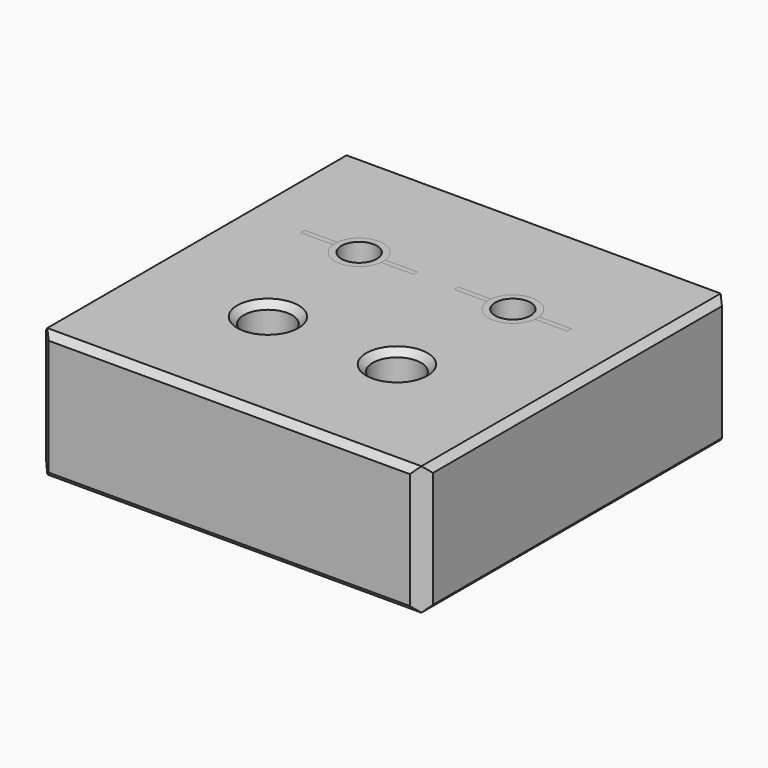
from build123d import *

# Parameters (mm, degrees)
F0_W        = 38.1
F0_H        = 76.2
F0_R        = 4.7625
F1_DEPTH    = 25.4
F2_SIZE     = 2.54
F3_SIZE     = 1.26999
F4_T1_DEPTH = 78.9220847894
F4_T3_DEPTH = 76.5265699849
F0_R_2      = 3.4925
F5_DEPTH    = 22.225
F6_DEPTH    = 22.225
F7_DEPTH    = 22.225
F8_SIZE     = 0.762
F8_2_SIZE   = 0.762
F9_SIZE2    = 1.6497783942
F9_SIZE     = 0.9525


# Not quite as in the source:
# - a fillet or chamfer that OpenCascade refuses, or shapes differently, is made with other operations: its cross-section is extruded or revolved along the edge and cut away or added
# - a fillet or chamfer is up to 0.001 mm smaller than in the source, because OpenCascade refuses the exact size


with BuildPart() as f1:
    # F0 (on Top) → F1 (new body)
    with BuildSketch(Plane.XY):
        with Locations((-19.05, 0)):
            Rectangle(F0_W, F0_H)
        with Locations((-12.7, -12.7)):
            Circle(F0_R, mode=Mode.SUBTRACT)
        with BuildLine():
            ThreePointArc((-19.8702153916, 13.3115481797), (-15.134886232, 17.5660481797), (-10.3995570724, 13.3115481797))
            Line((-10.3995570724, 13.3115481797), (-4.022386232, 13.3115481797))
            Line((-4.022386232, 13.3115481797), (-4.022386232, 12.2955481797))
            Line((-4.022386232, 12.2955481797), (-10.3995570724, 12.2955481797))
            ThreePointArc((-10.3995570724, 12.2955481797), (-15.134886232, 8.0410481797), (-19.8702153916, 12.2955481797))
            Line((-19.8702153916, 12.2955481797), (-26.247386232, 12.2955481797))
            Line((-26.247386232, 12.2955481797), (-26.247386232, 13.3115481797))
            Line((-26.247386232, 13.3115481797), (-19.8702153916, 13.3115481797))
        make_face(mode=Mode.SUBTRACT)
        with Locations((19.05, 0)):
            Rectangle(F0_W, F0_H)
        with Locations((12.7, -12.7)):
            Circle(F0_R, mode=Mode.SUBTRACT)
        with BuildLine():
            ThreePointArc((10.3995570724, 13.3115481797), (15.134886232, 17.5660481797), (19.8702153916, 13.3115481797))
            Line((19.8702153916, 13.3115481797), (26.247386232, 13.3115481797))
            Line((26.247386232, 13.3115481797), (26.247386232, 12.2955481797))
            Line((26.247386232, 12.2955481797), (19.8702153916, 12.2955481797))
            ThreePointArc((19.8702153916, 12.2955481797), (15.134886232, 8.0410481797), (10.3995570724, 12.2955481797))
            Line((10.3995570724, 12.2955481797), (4.022386232, 12.2955481797))
            Line((4.022386232, 12.2955481797), (4.022386232, 13.3115481797))
            Line((4.022386232, 13.3115481797), (10.3995570724, 13.3115481797))
        make_face(mode=Mode.SUBTRACT)
    extrude(amount=-F1_DEPTH)

    # F2
    f2_edges = [f1.edges().sort_by_distance(p)[0] for p in [
        (38.1, -38.1, -12.7),
        (38.1, 38.1, -12.7),
        (-38.1, -38.1, -12.7),
    ]]
    chamfer(f2_edges, length=F2_SIZE)

    # F3 (size 1.27 in the source; OpenCascade refuses exactly that, so slightly less here)
    f3_edges = [f1.edges().sort_by_distance(p)[0] for p in [
        (0, -38.1, 0),
        (-1.27, 38.1, 0),
        (38.1, 0, 0),
        (38.1, 0, -25.4),
        (0, -38.1, -25.4),
        (-1.27, 38.1, -25.4),
        (-38.1, 1.27, -25.4),
    ]]
    chamfer(f3_edges, length=F3_SIZE)

    # F4: chamfer of 1.27 on 4 edges, made by hand

    # F4_s2 → F4_t1 (cut)
    with BuildSketch(Plane.XZ.offset(-40.0960473947)):
        Polygon((-38.1, -1.27), (-36.83, 0), (-38.1, 0), align=None)
    extrude(amount=F4_T1_DEPTH, mode=Mode.SUBTRACT)

    # F4_s4 → F4_t3 (cut)
    with BuildSketch(Plane.XZ.offset(-39.5332849925)):
        Polygon((-38.1, -23.6039587758), (-37.7280256121, -24.5019843879), (-38.1, -24.13001), align=None)
    extrude(amount=F4_T3_DEPTH, mode=Mode.SUBTRACT)

    # F4_s5 → F4_t6 (revolve, cut)
    with BuildSketch(Plane.XZ.offset(12.7)):
        Polygon((-6.6675, 0), (-7.9375, -1.27), (-7.9375, 0), align=None)
    revolve(axis=Axis((-12.7, -12.7, 0), (0, 0, 1)), mode=Mode.SUBTRACT)

    # F4_s7 → F4_t8 (revolve, cut)
    with BuildSketch(Plane.XZ.offset(12.7)):
        Polygon((18.7325, 0), (17.4625, -1.27), (17.4625, 0), align=None)
    revolve(axis=Axis((12.7, -12.7, 0), (0, 0, 1)), mode=Mode.SUBTRACT)

    # F9
    f9_edges = [f1.edges().sort_by_distance(p)[0] for p in [
        (-23.058801, 12.295548, -25.4),
        (-26.247386, 12.803548, -25.4),
        (-23.058801, 13.311548, -25.4),
        (-7.210972, 12.295548, -25.4),
        (-4.022386, 12.803548, -25.4),
        (-7.210972, 13.311548, -25.4),
        (7.210972, 12.295548, -25.4),
        (4.022386, 12.803548, -25.4),
        (7.210972, 13.311548, -25.4),
        (23.058801, 12.295548, -25.4),
        (23.058801, 13.311548, -25.4),
        (26.247386, 12.803548, -25.4),
    ]]
    f9_side = f1.faces().sort_by_distance((0, -0.067575, -25.4))[0]
    chamfer(f9_edges, length=F9_SIZE, length2=F9_SIZE2, reference=f9_side)


with BuildPart() as f5:
    # F0 (on Top) → F5 (new body)
    with BuildSketch(Plane.XY):
        with BuildLine():
            ThreePointArc((19.8702153916, 12.2955481797), (19.8905886708, 12.549185125), (19.897386232, 12.8035481797))
            ThreePointArc((19.897386232, 12.8035481797), (19.8905886708, 13.0579112345), (19.8702153916, 13.3115481797))
            ThreePointArc((19.8702153916, 13.3115481797), (15.134886232, 17.5660481797), (10.3995570724, 13.3115481797))
            ThreePointArc((10.3995570724, 13.3115481797), (10.372386232, 12.8035481797), (10.3995570724, 12.2955481797))
            ThreePointArc((10.3995570724, 12.2955481797), (15.134886232, 8.0410481797), (19.8702153916, 12.2955481797))
        make_face()
        with Locations((15.134886232, 12.8035481797)):
            Circle(F0_R_2, mode=Mode.SUBTRACT)
    extrude(amount=-F5_DEPTH)

    # F8
    f8_edges = [f5.edges().sort_by_distance(p)[0] for p in [
        (11.642386, 12.803548, -22.225),
    ]]
    chamfer(f8_edges, length=F8_SIZE)


with BuildPart() as f5b:
    # F0 (on Top) → F5, piece 2 (new body)
    with BuildSketch(Plane.XY):
        with BuildLine():
            ThreePointArc((-10.3995570724, 12.2955481797), (-10.3791837932, 12.549185125), (-10.372386232, 12.8035481797))
            ThreePointArc((-10.372386232, 12.8035481797), (-10.3791837932, 13.0579112345), (-10.3995570724, 13.3115481797))
            ThreePointArc((-10.3995570724, 13.3115481797), (-15.134886232, 17.5660481797), (-19.8702153916, 13.3115481797))
            ThreePointArc((-19.8702153916, 13.3115481797), (-19.897386232, 12.8035481797), (-19.8702153916, 12.2955481797))
            ThreePointArc((-19.8702153916, 12.2955481797), (-15.134886232, 8.0410481797), (-10.3995570724, 12.2955481797))
        make_face()
        with Locations((-15.134886232, 12.8035481797)):
            Circle(F0_R_2, mode=Mode.SUBTRACT)
    extrude(amount=-F5_DEPTH)

    # F8#2
    f8_2_edges = [f5b.edges().sort_by_distance(p)[0] for p in [
        (-18.627386, 12.803548, -22.225),
    ]]
    chamfer(f8_2_edges, length=F8_2_SIZE)


with BuildPart() as f6:
    # F0 (on Top) → F6 (new body)
    with BuildSketch(Plane.XY):
        with BuildLine():
            ThreePointArc((-10.3995570724, 13.3115481797), (-10.3791837932, 13.0579112345), (-10.372386232, 12.8035481797))
            ThreePointArc((-10.372386232, 12.8035481797), (-10.3791837932, 12.549185125), (-10.3995570724, 12.2955481797))
            Line((-10.3995570724, 12.2955481797), (-4.022386232, 12.2955481797))
            Line((-4.022386232, 12.2955481797), (-4.022386232, 13.3115481797))
            Line((-4.022386232, 13.3115481797), (-10.3995570724, 13.3115481797))
        make_face()
    extrude(amount=-F6_DEPTH)


with BuildPart() as f6b:
    # F0 (on Top) → F6, piece 2 (new body)
    with BuildSketch(Plane.XY):
        with BuildLine():
            ThreePointArc((-19.8702153916, 12.2955481797), (-19.897386232, 12.8035481797), (-19.8702153916, 13.3115481797))
            Line((-19.8702153916, 13.3115481797), (-26.247386232, 13.3115481797))
            Line((-26.247386232, 13.3115481797), (-26.247386232, 12.2955481797))
            Line((-26.247386232, 12.2955481797), (-19.8702153916, 12.2955481797))
        make_face()
    extrude(amount=-F6_DEPTH)


with BuildPart() as f7:
    # F0 (on Top) → F7 (new body)
    with BuildSketch(Plane.XY):
        with BuildLine():
            ThreePointArc((10.3995570724, 12.2955481797), (10.372386232, 12.8035481797), (10.3995570724, 13.3115481797))
            Line((10.3995570724, 13.3115481797), (4.022386232, 13.3115481797))
            Line((4.022386232, 13.3115481797), (4.022386232, 12.2955481797))
            Line((4.022386232, 12.2955481797), (10.3995570724, 12.2955481797))
        make_face()
    extrude(amount=-F7_DEPTH)


with BuildPart() as f7b:
    # F0 (on Top) → F7, piece 2 (new body)
    with BuildSketch(Plane.XY):
        with BuildLine():
            ThreePointArc((19.8702153916, 13.3115481797), (19.8905886708, 13.0579112345), (19.897386232, 12.8035481797))
            ThreePointArc((19.897386232, 12.8035481797), (19.8905886708, 12.549185125), (19.8702153916, 12.2955481797))
            Line((19.8702153916, 12.2955481797), (26.247386232, 12.2955481797))
            Line((26.247386232, 12.2955481797), (26.247386232, 13.3115481797))
            Line((26.247386232, 13.3115481797), (19.8702153916, 13.3115481797))
        make_face()
    extrude(amount=-F7_DEPTH)


solid = Compound([f1.part, f5.part, f5b.part, f6.part, f6b.part, f7.part, f7b.part])
